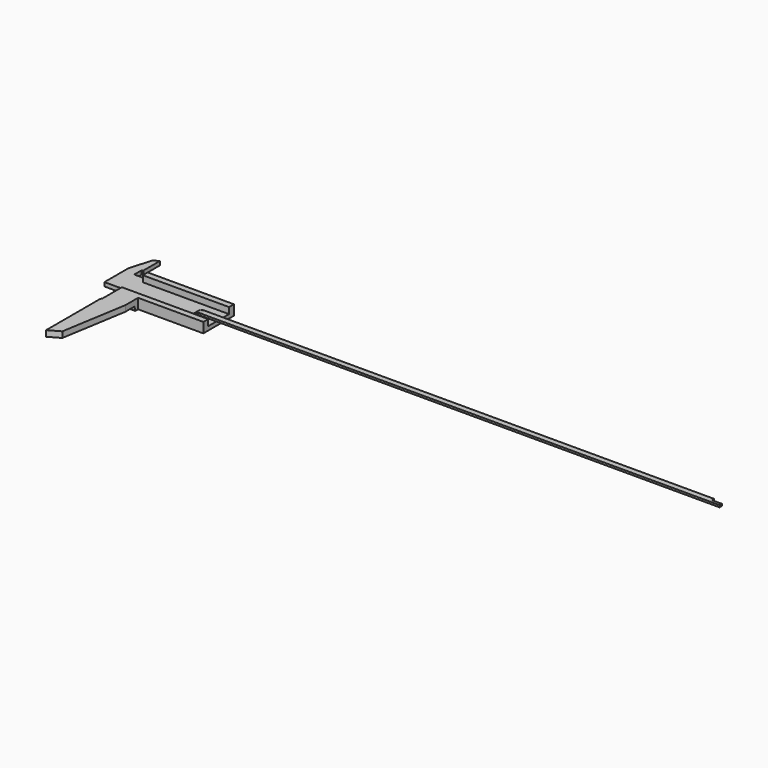
from build123d import *

# Parameters (mm, degrees)
F2_DEPTH     = 6.604
F4_W         = 17.018
F4_H         = 5.5950877881
F5_DEPTH     = 71.6798
F6_W         = 16.355678454
F6_H         = 4.3095059386
F7_DEPTH     = 44.9793598678
F9_DEPTH     = 56.897
F10_W        = 342.8717973226
F10_H        = 3.7084
F11_DEPTH    = 1.27
F12_T1_DEPTH = 3.7084
F14_DEPTH    = 4.065


# Not quite as in the source:
# - a fillet or chamfer that OpenCascade refuses, or shapes differently, is made with other operations: its cross-section is extruded or revolved along the edge and cut away or added


with BuildPart() as f2:
    # F1 (on Top) → F2 (new body)
    with BuildSketch(Plane.XY):
        Polygon((80.7733850724, 0), (80.7733850724, 24.9428), (15.7493850724, 24.9428), (15.7493850724, 30.8864), (16.6319306082, 31.5163598678), (16.6319306082, 44.9783598678), (13.1174201358, 42.4697068149), (9.0945850724, 28.2448), (9.0945850724, 8.9408), (24.4869850724, 8.9408), (24.4869850724, -11.8872), (23.8773850724, -13.1876401322), (23.8773850724, -57.1296401322), (31.1824725433, -53.0194550947), (38.2029850724, -10.414), (38.2029850724, 0), align=None)
    extrude(amount=F2_DEPTH)

    # F4 (on face) → F5 (cut, through all)
    with BuildSketch(Plane(origin=(9.0945850724, 0, 0), x_dir=(0, -1, 0), z_dir=(-1, 0, 0))):
        with Locations((-12.4714, 5.3375438941)):
            Rectangle(F4_W, F4_H)
    extrude(amount=-F5_DEPTH, mode=Mode.SUBTRACT)

    # F6 (on Front) → F7 (cut, through all)
    with BuildSketch(Plane.XZ):
        with Locations((16.3091458454, 4.6947529693)):
            Rectangle(F6_W, F6_H)
    extrude(amount=-F7_DEPTH, mode=Mode.SUBTRACT)

    # F8 (on face) → F9 (cut, through all)
    with BuildSketch(Plane(origin=(23.8773850724, 0, 0), x_dir=(0, -1, 0), z_dir=(-1, 0, 0))):
        Polygon((57.1296401322, -1.4798081247), (57.1296401322, 2.794), (2.9003161471, 2.794), (2.032, -1.4798081247), align=None)
    extrude(amount=-F9_DEPTH, mode=Mode.SUBTRACT)

    # F10 (on face) → F11 (join)
    with BuildSketch(Plane.XY.offset(2.54)):
        with Locations((237.7086864111, 12.4714)):
            Rectangle(F10_W, F10_H)
    extrude(amount=F11_DEPTH)

    # F12: fillet of radius 6.35 on 1 edges, made by hand

    # F12_s2 → F12_t1 (cut)
    with BuildSketch(Plane.XZ.offset(-14.3256)):
        with BuildLine():
            ThreePointArc((66.2727877498, 2.54), (68.0747414356, 3.4841389426), (70.0827877498, 3.81))
            Line((70.0827877498, 3.81), (66.2727877498, 3.81))
            Line((66.2727877498, 3.81), (66.2727877498, 2.54))
        make_face()
    extrude(amount=F12_T1_DEPTH, mode=Mode.SUBTRACT)

    # F13 (on face) → F14 (cut, through all)
    with BuildSketch(Plane(origin=(0, 0, 2.54), x_dir=(1, 0, 0), z_dir=(0, 0, -1))):
        with BuildLine():
            ThreePointArc((403.4869184795, -12.5476), (402.7459176611, -12.8545325887), (402.4389850724, -13.5955334071))
            Line((402.4389850724, -13.5955334071), (402.4389850724, -14.3256))
            Line((402.4389850724, -14.3256), (409.480124712, -15.0942075998))
            Line((409.480124712, -15.0942075998), (409.1445850724, -12.5476))
            Line((409.1445850724, -12.5476), (403.4869184795, -12.5476))
        make_face()
    extrude(amount=-F14_DEPTH, mode=Mode.SUBTRACT)


solid = f2.part
